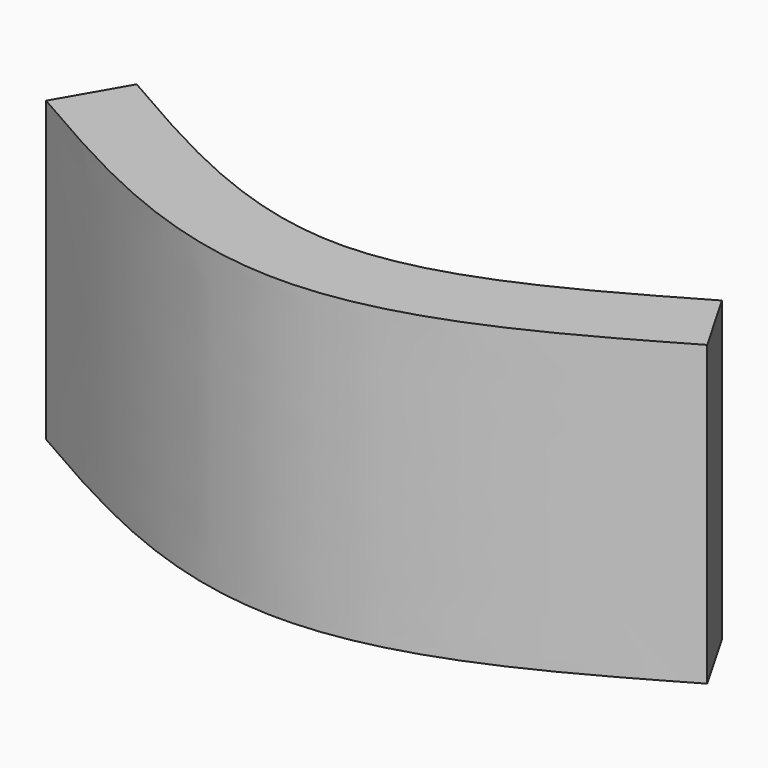
from build123d import *

# Parameters (mm, degrees)
F1_DEPTH = 67.31


# Not quite as in the source:
# - the dataset's text gives a spline's control points without its knots; the knots are read off the source's solid


with BuildPart() as f1:
    # F0 (on Top) → F1 (new body)
    with BuildSketch(Plane.XY):
        with BuildLine():
            add(Edge.make_bspline(
                [(-66.04, 25.4), (-44.0266666667, 12.7), (0, -12.7), (44.0266666667, 12.7), (66.04, 25.4)],
                knots=[0, 0, 0, 0, 0.5, 1, 1, 1, 1], degree=3))
            Line((-66.04, 25.4), (-74.6077414651, 10.5492481272))
            add(Edge.make_bspline(
                [(-74.6077414651, 10.5492481272), (-71.8560747984, 8.9617481272), (-66.2861722031, 5.7480427564), (-57.724560048, 0.9615668395), (-48.9347700683, -3.6367958027), (-39.8807925782, -7.8853107319), (-32.0742809117, -10.9875301018), (-25.6442375738, -13.1047930023), (-20.7230725464, -14.4812886294), (-15.6987085879, -15.6150662473), (-11.4242321111, -16.3292183153), (-7.9537726238, -16.7440164926), (-5.3260159043, -16.9721840593), (-2.6763709835, -17.1127600702), (0, -17.1611199649), (2.6763709835, -17.1127600702), (5.3260159043, -16.9721840593), (7.9537726238, -16.7440164926), (11.4242321111, -16.3292183153), (15.6987085879, -15.6150662473), (20.7230725464, -14.4812886294), (25.6442375738, -13.1047930023), (32.0742809117, -10.9875301018), (39.8807925782, -7.8853107319), (48.9347700683, -3.6367958027), (57.724560048, 0.9615668395), (66.2861722031, 5.7480427564), (71.8560747984, 8.9617481272), (74.6077414651, 10.5492481272)],
                knots=[0, 0, 0, 0, 0.0625, 0.125, 0.1875, 0.25, 0.3125, 0.34375, 0.375, 0.40625, 0.4375, 0.453125, 0.46875, 0.484375, 0.5, 0.515625, 0.53125, 0.546875, 0.5625, 0.59375, 0.625, 0.65625, 0.6875, 0.75, 0.8125, 0.875, 0.9375, 1, 1, 1, 1], degree=3))
            Line((74.6077414651, 10.5492481272), (66.04, 25.4))
        make_face()
    extrude(amount=F1_DEPTH)


solid = f1.part
